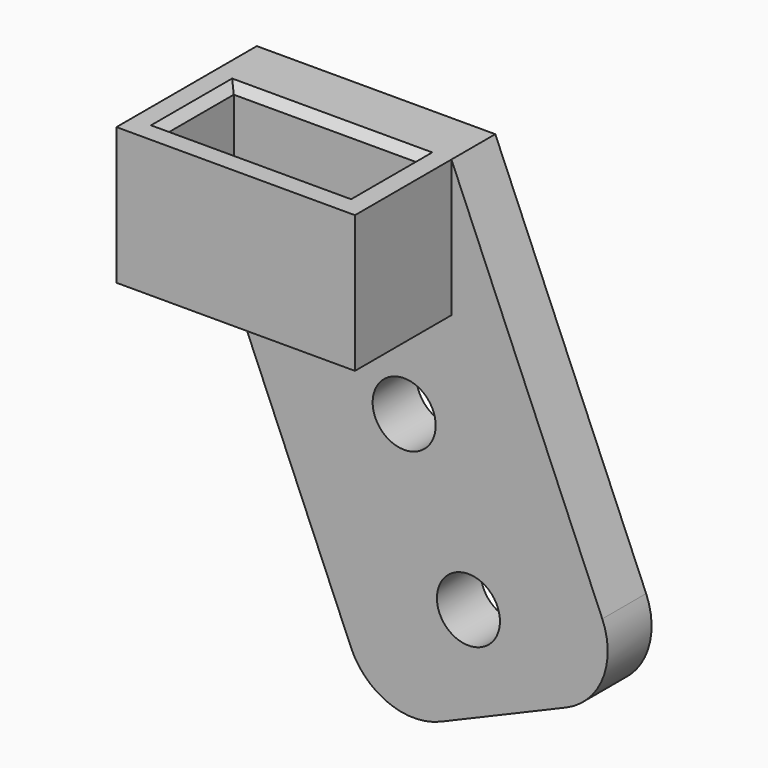
from build123d import *

# Parameters (mm, degrees)
F0_W     = 17.4
F0_H     = 8.8
F0_W_2   = 13.4
F0_H_2   = 6.2
F1_DEPTH = 10
F2_W     = 17.4
F2_H     = 10
F3_DEPTH = 4
F4_D     = 4.6
F4_DEPTH = 10
F4_TIP   = 1.3819794238
F5_R     = 5
F6_SIZE  = 0.6


# Not quite as in the source:
# - a feature names something its author has since deleted; it is built from what else it names


with BuildPart() as f1:
    # F0 (on Top) → F1 (new body)
    with BuildSketch(Plane.XY):
        with Locations((-5.3887722373, 2.3212898893)):
            Rectangle(F0_W, F0_H)
        with Locations((-5.3887722373, 3.0212898893)):
            Rectangle(F0_W_2, F0_H_2, mode=Mode.SUBTRACT)
    extrude(amount=F1_DEPTH)

    # F2 (on face) → F3 (join)
    with BuildSketch(Plane(origin=(0, 6.7212898893, 0), x_dir=(-1, 0, 0), z_dir=(0, 1, 0))):
        with Locations((5.3887722373, 5)):
            Rectangle(F2_W, F2_H)
        Polygon((-3.3112277627, 0), (-3.3112277627, 10), (-16.2704663397, -20.530052861), (2.069760485, -28.3150172716), (14.0887722373, 0), align=None)
    extrude(amount=F3_DEPTH)

    # F4
    with Locations(Plane(origin=(0, 6.7212898893, 0), x_dir=(-1, 0, 0), z_dir=(0, -1, 0))):
        with Locations((0.1372122432, 7.4690311061), (-4.5515612986, 18.5150893475)):
            Hole(F4_D / 2, depth=F4_DEPTH)
            with Locations((0, 0, -(F4_DEPTH + F4_TIP / 2))):  # 118° drill point
                Cone(0, F4_D / 2, F4_TIP, mode=Mode.SUBTRACT)

    # F5
    f5_edges = [f1.edges().sort_by_distance(p)[0] for p in [
        (16.270466, 8.72129, -20.530053),
        (-2.06976, 8.72129, -28.315017),
    ]]
    fillet(f5_edges, radius=F5_R)

    # F6
    f6_edges = [f1.edges().sort_by_distance(p)[0] for p in [
        (-5.388772, 6.12129, 10),
        (1.311228, 3.02129, 10),
        (-12.088772, 3.02129, 10),
        (-5.388772, -0.07871, 10),
    ]]
    chamfer(f6_edges, length=F6_SIZE)


solid = f1.part
